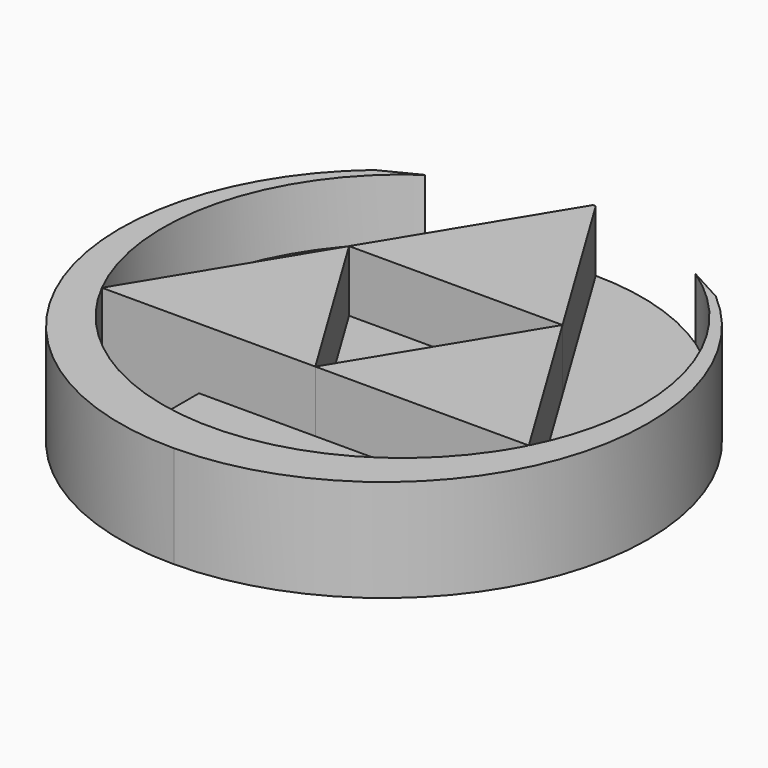
from build123d import *

# Parameters (mm, degrees)
F1_DEPTH = 12.7
F2_DEPTH = 5.08


# Not quite as in the source:
# - a feature names something its author has since deleted; it is built from what else it names


with BuildPart() as f1:
    # F0 (on Top) → F1 (new body)
    with BuildSketch(Plane.XY):
        with BuildLine():
            Line((-0.7304638443, 17.6570977744), (-13.8243847458, 39.1909619838))
            ThreePointArc((-13.8243847458, 39.1909619838), (-14.0022787977, 39.1914928804), (-14.1801728496, 39.1909619839))
            Line((-14.1801728496, 39.1909619839), (-27.2740937544, 17.6570977744))
            Line((-27.2740937544, 17.6570977744), (-0.7304638443, 17.6570977744))
        make_face()
    extrude(amount=F1_DEPTH)


with BuildPart() as f1b:
    # F0 (on Top) → F1, piece 2 (new body)
    with BuildSketch(Plane.XY):
        Polygon((-14.0052981097, -4.1693255842), (-27.2740937544, 17.6570977744), (-40.5459087111, -4.1693255842), (-28.4659001209, -4.1693255842), (-24.5637800544, -4.1693255842), align=None)
    extrude(amount=F1_DEPTH)


with BuildPart() as f1c:
    # F0 (on Top) → F1, piece 3 (new body)
    with BuildSketch(Plane.XY):
        Polygon((4.6093779556, -4.1693255842), (12.5413511092, -4.1693255842), (-0.7304638443, 17.6570977744), (-14.002278801, -4.1693255842), (-3.4407775408, -4.1693255842), align=None)
    extrude(amount=F1_DEPTH)


with BuildPart() as f1d:
    # F0 (on Top) → F1, piece 4 (new body)
    with BuildSketch(Plane.XY):
        with BuildLine():
            ThreePointArc((2.6267673161, 34.121311843), (12.3031850523, 23.3991896828), (15.8025652754, 9.386648804))
            ThreePointArc((15.8025652754, 9.386648804), (14.9770861572, 2.4206501647), (12.5463739719, -4.1594859348))
            Line((12.5463739719, -4.1594859348), (12.546375676, -4.1742923649))
            Line((12.546375676, -4.1742923649), (12.5388143231, -4.1742916575))
            ThreePointArc((12.5388143231, -4.1742916575), (11.6934665545, -5.7149206854), (10.7587911193, -7.2030512181))
            ThreePointArc((10.7587911193, -7.2030512181), (-7.0067815574, -19.5856094569), (-28.4652345808, -16.6738891899))
            ThreePointArc((-28.4652345808, -16.6738891899), (-35.4376711517, -11.3221098549), (-40.5459087111, -4.1693255842))
            ThreePointArc((-40.5459087111, -4.1693255842), (-42.8906697283, 16.7207881569), (-30.8650428104, 33.9625703611))
            Line((-30.8650428104, 33.9625703611), (-35.3768183074, 31.682918978))
            ThreePointArc((-35.3768183074, 31.682918978), (-44.9205686415, -4.7129685745), (-14.0022787977, -26.1559896842))
            ThreePointArc((-14.0022787977, -26.1559896842), (16.6955901847, -4.587967654), (7.1059333978, 31.682918978))
            Line((7.1059333978, 31.682918978), (2.6267673161, 34.121311843))
        make_face()
    extrude(amount=F1_DEPTH)


with BuildPart() as f2:
    # F0 (on Top) → F2 (new body)
    with BuildSketch(Plane.XY):
        Polygon((-14.002278801, -4.1693255842), (-0.7304638443, 17.6570977744), (-27.2740937544, 17.6570977744), (-14.0052981097, -4.1693255842), align=None)
    extrude(amount=F2_DEPTH)


with BuildPart() as f2b:
    # F0 (on Top) → F2, piece 2 (new body)
    with BuildSketch(Plane.XY):
        with BuildLine():
            ThreePointArc((-28.4652345808, -16.6738891899), (-7.0067815574, -19.5856094569), (10.7587911193, -7.2030512181))
            Line((10.7587911193, -7.2030512181), (4.6179422563, -4.1735506603))
            Line((4.6179422563, -4.1735506603), (-3.4407775408, -4.1727967674))
            Line((-3.4407775408, -4.1727967674), (-14.0037886271, -4.1718085983))
            Line((-14.0037886271, -4.1718085983), (-24.5637800544, -4.1708207116))
            Line((-24.5637800544, -4.1708207116), (-28.4659000607, -4.1704556684))
            Line((-28.4659000607, -4.1704556684), (-28.4652345808, -16.6738891899))
        make_face()
    extrude(amount=F2_DEPTH)


with BuildPart() as f2c:
    # F0 (on Top) → F2, piece 3 (new body)
    with BuildSketch(Plane.XY):
        with BuildLine():
            Line((-27.2740937544, 17.6570977744), (-14.1801728496, 39.1909619839))
            ThreePointArc((-14.1801728496, 39.1909619839), (-22.9146312684, 37.8277933645), (-30.8650428104, 33.9625703611))
            ThreePointArc((-30.8650428104, 33.9625703611), (-42.8906697283, 16.7207881569), (-40.5459087111, -4.1693255842))
            Line((-40.5459087111, -4.1693255842), (-27.2740937544, 17.6570977744))
        make_face()
    extrude(amount=F2_DEPTH)


with BuildPart() as f2d:
    # F0 (on Top) → F2, piece 4 (new body)
    with BuildSketch(Plane.XY):
        with BuildLine():
            ThreePointArc((12.5463739719, -4.1594859348), (14.9770861572, 2.4206501647), (15.8025652754, 9.386648804))
            ThreePointArc((15.8025652754, 9.386648804), (12.3031850523, 23.3991896828), (2.6267673161, 34.121311843))
            ThreePointArc((2.6267673161, 34.121311843), (-5.2248277116, 37.8697154014), (-13.8243847458, 39.1909619838))
            Line((-13.8243847458, 39.1909619838), (-0.7304638443, 17.6570977744))
            Line((-0.7304638443, 17.6570977744), (12.5413511092, -4.1693255842))
            ThreePointArc((12.5413511092, -4.1693255842), (12.5438629964, -4.1644059922), (12.5463739719, -4.1594859348))
        make_face()
    extrude(amount=F2_DEPTH)


solid = Compound([f1.part, f1b.part, f1c.part, f1d.part, f2.part, f2b.part, f2c.part, f2d.part])
